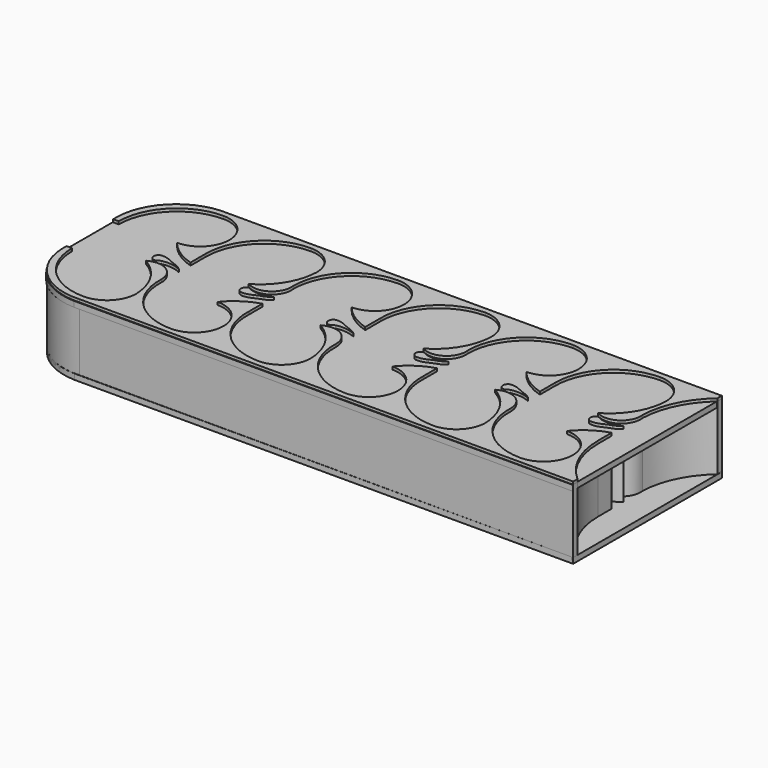
from build123d import *

# Parameters (mm, degrees)
F1_DEPTH = 12
F3_DEPTH = 0.5
F5_DEPTH = 1
F6_DEPTH = 0.5
F7_DEPTH = 0.5


# Not quite as in the source:
# - ends of sketch curves that miss each other by under 0.0002 mm in the source are joined


with BuildPart() as f1:
    # F0 (on Top) → F1 (new body)
    with BuildSketch(Plane.XY):
        with BuildLine():
            Line((-4.0578052044, 17.8321947956), (-3.0578052044, 17.8321947956))
            ThreePointArc((-3.0578052044, 17.8321947956), (0, 25.2143895912), (7.3821947956, 28.2721947956))
            ThreePointArc((7.3821947956, 28.2721947956), (12.6021947956, 23.0521947956), (7.3821947956, 17.8321947956))
            ThreePointArc((7.3821947956, 17.8321947956), (9.7268158019, 15.6873529518), (12.6080603792, 14.3471947956))
            Line((12.6080603792, 14.3471947956), (12.6057125985, 17.8321947956))
            ThreePointArc((12.6057125985, 17.8321947956), (15.663517803, 25.2143895912), (23.0457125985, 28.2721947956))
            ThreePointArc((23.0457125985, 28.2721947956), (26.735512433, 26.74199463), (28.2657125985, 23.0521947956))
            ThreePointArc((28.2657125985, 23.0521947956), (26.7848210646, 18.0226188401), (23.0457125985, 14.3471947956))
            ThreePointArc((23.0457125985, 14.3471947956), (26.7558378252, 14.4434003756), (28.2692304015, 17.8321947956))
            ThreePointArc((28.2692304015, 17.8321947956), (31.3266820271, 25.2140360912), (38.7082304015, 28.2721948435))
            ThreePointArc((38.7082304015, 28.2721948435), (38.7087304015, 28.2721948794), (38.7092304015, 28.2721948914))
            ThreePointArc((38.7092304015, 28.2721948914), (43.9282304015, 23.0521947956), (38.7092304015, 17.8321948914))
            ThreePointArc((38.7092304015, 17.8321948914), (38.7087304015, 17.8321948195), (38.7082304015, 17.8321947956))
            ThreePointArc((38.7082304015, 17.8321947956), (41.0528514078, 15.6873529518), (43.9340959851, 14.3471947956))
            Line((43.9340959851, 14.3471947956), (43.9317482044, 17.8321947956))
            ThreePointArc((43.9317482044, 17.8321947956), (46.989553375, 25.2143896531), (54.3717482044, 28.2721948914))
            ThreePointArc((54.3717482044, 28.2721948914), (58.0616124348, 26.7423520877), (59.5907482044, 23.0521947956))
            ThreePointArc((59.5907482044, 23.0521947956), (58.1098566705, 18.0226188401), (54.3707482044, 14.3471947956))
            ThreePointArc((54.3707482044, 14.3471947956), (58.0808734311, 14.4434003756), (59.5942660074, 17.8321947956))
            ThreePointArc((59.5942660074, 17.8321947956), (62.651717633, 25.2140360912), (70.0332660074, 28.2721948435))
            ThreePointArc((70.0332660074, 28.2721948435), (70.0337660074, 28.2721948794), (70.0342660074, 28.2721948914))
            ThreePointArc((70.0342660074, 28.2721948914), (75.2532660074, 23.0521947956), (70.0342660074, 17.8321948914))
            ThreePointArc((70.0342660074, 17.8321948914), (70.0337660074, 17.8321948195), (70.0332660074, 17.8321947956))
            ThreePointArc((70.0332660074, 17.8321947956), (72.3778870137, 15.6873529518), (75.259131591, 14.3471947956))
            Line((75.259131591, 14.3471947956), (75.2567838104, 17.8321947956))
            ThreePointArc((75.2567838104, 17.8321947956), (78.3145889809, 25.2143896531), (85.6967838104, 28.2721948914))
            ThreePointArc((85.6967838104, 28.2721948914), (89.3869966698, 26.74270065), (90.9157838104, 23.0521947956))
            ThreePointArc((90.9157838104, 23.0521947956), (89.4348922764, 18.0226188401), (85.6957838104, 14.3471947956))
            ThreePointArc((85.6957838104, 14.3471947956), (89.405909037, 14.4434003756), (90.9193016133, 17.8321947956))
            ThreePointArc((90.9193016133, 17.8321947956), (92.3441007337, 23.5750026665), (95.9421947956, 28.2721947956))
            Line((95.9421947956, 28.2721947956), (95.9421947956, 29.2721947956))
            Line((95.9421947956, 29.2721947956), (7.3821947956, 29.2721947956))
            ThreePointArc((7.3821947956, 29.2721947956), (-0.5342205883, 26.4589947948), (-4.0578052044, 18.8321947956))
            Line((-4.0578052044, 18.8321947956), (-4.0578052044, 17.8321947956))
        make_face()
    extrude(amount=F1_DEPTH)


with BuildPart() as f1b:
    # F0 (on Top) → F1, piece 2 (new body)
    with BuildSketch(Plane.XY):
        with BuildLine():
            Line((-3.0578052044, 7.3821947956), (-4.0578052044, 7.3821947956))
            Line((-4.0578052044, 7.3821947956), (-4.0578052044, 6.3821947956))
            ThreePointArc((-4.0578052044, 6.3821947956), (-0.532322416, -1.242525214), (7.3821947956, -4.0578052044))
            Line((7.3821947956, -4.0578052044), (95.9421947956, -4.0578052044))
            Line((95.9421947956, -4.0578052044), (95.9421947956, -3.0578052044))
            ThreePointArc((95.9421947956, -3.0578052044), (92.2352959866, 1.8486137013), (90.9193016133, 7.8554601342))
            Line((90.9193016133, 7.8554601342), (90.9193016133, 10.8671947956))
            ThreePointArc((90.9193016133, 10.8671947956), (88.0393184071, 9.5267247614), (85.6957838104, 7.3821947956))
            ThreePointArc((85.6957838104, 7.3821947956), (90.9157838104, 2.1621947956), (85.6957838104, -3.0578052045))
            ThreePointArc((85.6957838104, -3.0578052045), (85.690917339, -3.0578086106), (85.6860508666, -3.0578097483))
            ThreePointArc((85.6860508666, -3.0578097483), (78.1383828537, 0.1692592999), (75.2567838104, 7.8554601342))
            ThreePointArc((75.2567838104, 7.8554601342), (73.515024019, 10.8702438705), (70.0332660074, 10.8671947956))
            ThreePointArc((70.0332660074, 10.8671947956), (73.7723744735, 7.1917707511), (75.2532660074, 2.1621947956))
            ThreePointArc((75.2532660074, 2.1621947956), (73.7199871381, -1.5314121329), (70.0235330637, -3.0578142782))
            ThreePointArc((70.0235330637, -3.0578142782), (62.4758650508, 0.1692592999), (59.5942660074, 7.8554601342))
            Line((59.5942660074, 7.8554601342), (59.5942660074, 10.8671947956))
            ThreePointArc((59.5942660074, 10.8671947956), (56.7142828012, 9.5267247614), (54.3707482044, 7.3821947956))
            ThreePointArc((54.3707482044, 7.3821947956), (59.5907482044, 2.1621947956), (54.3707482044, -3.0578052044))
            ThreePointArc((54.3707482044, -3.0578052044), (54.3658817331, -3.0578086106), (54.3610152607, -3.0578097483))
            ThreePointArc((54.3610152607, -3.0578097483), (46.8133472478, 0.1692592999), (43.9317482044, 7.8554601342))
            ThreePointArc((43.9317482044, 7.8554601342), (42.1899884131, 10.8702438705), (38.7082304015, 10.8671947956))
            ThreePointArc((38.7082304015, 10.8671947956), (42.4473388676, 7.1917707511), (43.9282304015, 2.1621947956))
            ThreePointArc((43.9282304015, 2.1621947956), (42.3950425449, -1.5315033151), (38.6984974577, -3.0578142782))
            ThreePointArc((38.6984974577, -3.0578142782), (31.1508294449, 0.1692592999), (28.2692304015, 7.8554601342))
            Line((28.2692304015, 7.8554601342), (28.2692304015, 10.8671947956))
            ThreePointArc((28.2692304015, 10.8671947956), (25.3892471953, 9.5267247614), (23.0457125985, 7.3821947956))
            ThreePointArc((23.0457125985, 7.3821947956), (26.7368099963, 5.8532921934), (28.2657125985, 2.1621947956))
            ThreePointArc((28.2657125985, 2.1621947956), (26.7368099963, -1.5289026022), (23.0457125985, -3.0578052044))
            ThreePointArc((23.0457125985, -3.0578052044), (23.0403460829, -3.0578093467), (23.0349795658, -3.0578107304))
            ThreePointArc((23.0349795658, -3.0578107304), (15.487310875, 0.1692583362), (12.6057125985, 7.8554604215))
            ThreePointArc((12.6057125985, 7.8554604215), (10.8639528072, 10.8702441579), (7.3821947956, 10.8671950829))
            ThreePointArc((7.3821947956, 10.8671950829), (11.1213033303, 7.1917709136), (12.6021947956, 2.1621947956))
            ThreePointArc((12.6021947956, 2.1621947956), (11.0722754954, -1.5278859042), (7.3821947956, -3.0578052044))
            ThreePointArc((7.3821947956, -3.0578052044), (0, 0), (-3.0578052044, 7.3821947956))
        make_face()
    extrude(amount=F1_DEPTH)


with BuildPart() as f1c:
    # F0 (on Top) → F1, piece 3 (new body)
    with BuildSketch(Plane.XY):
        with BuildLine():
            ThreePointArc((9.9950144552, 13.0421947956), (9.1526392653, 13.3739527192), (8.2531947956, 13.4771947956))
            ThreePointArc((8.2531947956, 13.4771947956), (7.6380119976, 13.2223777968), (7.3831947956, 12.6071950829))
            ThreePointArc((7.3831947956, 12.6071950829), (7.6380117944, 11.9920119976), (8.2531947956, 11.7371947956))
            ThreePointArc((8.2531947956, 11.7371947956), (8.6734073917, 11.9853047468), (9.1241947956, 12.1721947956))
            ThreePointArc((9.1241947956, 12.1721947956), (10.9028963095, 12.2560700802), (12.6062995437, 11.7371947956))
            ThreePointArc((12.6062995437, 11.7371947956), (11.983253552, 12.2040695598), (11.2720043124, 12.5207442706))
            ThreePointArc((11.2720043124, 12.5207442706), (10.6248880882, 12.7603566825), (9.9950144552, 13.0421947956))
        make_face()
    extrude(amount=F1_DEPTH)


with BuildPart() as f1d:
    # F0 (on Top) → F1, piece 4 (new body)
    with BuildSketch(Plane.XY):
        with BuildLine():
            ThreePointArc((24.7867125985, 13.0421947956), (24.3359251946, 13.2290848443), (23.9157125985, 13.4771947956))
            ThreePointArc((23.9157125985, 13.4771947956), (23.3005296989, 13.2223776952), (23.0457125985, 12.6071947956))
            ThreePointArc((23.0457125985, 12.6071947956), (23.3005296989, 11.992011896), (23.9157125985, 11.7371947956))
            ThreePointArc((23.9157125985, 11.7371947956), (24.8152501168, 11.8404135156), (25.6577125985, 12.1721947956))
            ThreePointArc((25.6577125985, 12.1721947956), (26.2876842061, 12.4540520233), (26.9349016865, 12.6936710042))
            ThreePointArc((26.9349016865, 12.6936710042), (27.6465662844, 13.0102546924), (28.269991237, 13.4771947956))
            ThreePointArc((28.269991237, 13.4771947956), (26.5660143275, 12.9581116528), (24.7867125985, 13.0421947956))
        make_face()
    extrude(amount=F1_DEPTH)


with BuildPart() as f1e:
    # F0 (on Top) → F1, piece 5 (new body)
    with BuildSketch(Plane.XY):
        with BuildLine():
            ThreePointArc((41.3200500611, 13.0421947956), (40.4776748712, 13.3739527192), (39.5782304015, 13.4771947956))
            ThreePointArc((39.5782304015, 13.4771947956), (38.9630475019, 13.2223776952), (38.7082304015, 12.6071947956))
            ThreePointArc((38.7082304015, 12.6071947956), (38.9630475019, 11.992011896), (39.5782304015, 11.7371947956))
            ThreePointArc((39.5782304015, 11.7371947956), (39.9984429976, 11.9853047468), (40.4492304015, 12.1721947956))
            ThreePointArc((40.4492304015, 12.1721947956), (42.2279319155, 12.2560700802), (43.9313351496, 11.7371947956))
            ThreePointArc((43.9313351496, 11.7371947956), (43.3082891579, 12.2040695598), (42.5970399183, 12.5207442706))
            ThreePointArc((42.5970399183, 12.5207442706), (41.9499236941, 12.7603566825), (41.3200500611, 13.0421947956))
        make_face()
    extrude(amount=F1_DEPTH)


with BuildPart() as f1f:
    # F0 (on Top) → F1, piece 6 (new body)
    with BuildSketch(Plane.XY):
        with BuildLine():
            ThreePointArc((56.1117482044, 13.0421947956), (55.6609608006, 13.2290848443), (55.2407482044, 13.4771947956))
            ThreePointArc((55.2407482044, 13.4771947956), (54.6255653048, 13.2223776952), (54.3707482044, 12.6071947956))
            ThreePointArc((54.3707482044, 12.6071947956), (54.6255653048, 11.992011896), (55.2407482044, 11.7371947956))
            ThreePointArc((55.2407482044, 11.7371947956), (56.1402857227, 11.8404135156), (56.9827482044, 12.1721947956))
            ThreePointArc((56.9827482044, 12.1721947956), (57.612719812, 12.4540520233), (58.2599372924, 12.6936710042))
            ThreePointArc((58.2599372924, 12.6936710042), (58.9716018903, 13.0102546924), (59.5950268429, 13.4771947956))
            ThreePointArc((59.5950268429, 13.4771947956), (57.8910499334, 12.9581116528), (56.1117482044, 13.0421947956))
        make_face()
    extrude(amount=F1_DEPTH)


with BuildPart() as f1g:
    # F0 (on Top) → F1, piece 7 (new body)
    with BuildSketch(Plane.XY):
        with BuildLine():
            ThreePointArc((72.645085667, 13.0421947956), (71.8027104771, 13.3739527192), (70.9032660074, 13.4771947956))
            ThreePointArc((70.9032660074, 13.4771947956), (70.2880831078, 13.2223776952), (70.0332660074, 12.6071947956))
            ThreePointArc((70.0332660074, 12.6071947956), (70.2880831078, 11.992011896), (70.9032660074, 11.7371947956))
            ThreePointArc((70.9032660074, 11.7371947956), (71.3234786035, 11.9853047468), (71.7742660074, 12.1721947956))
            ThreePointArc((71.7742660074, 12.1721947956), (73.5529675214, 12.2560700802), (75.2563707555, 11.7371947956))
            ThreePointArc((75.2563707555, 11.7371947956), (74.6333247638, 12.2040695598), (73.9220755242, 12.5207442706))
            ThreePointArc((73.9220755242, 12.5207442706), (73.2749593, 12.7603566825), (72.645085667, 13.0421947956))
        make_face()
    extrude(amount=F1_DEPTH)


with BuildPart() as f1h:
    # F0 (on Top) → F1, piece 8 (new body)
    with BuildSketch(Plane.XY):
        with BuildLine():
            ThreePointArc((87.4367838104, 13.0421947956), (86.9859964065, 13.2290848443), (86.5657838104, 13.4771947956))
            ThreePointArc((86.5657838104, 13.4771947956), (85.9506009107, 13.2223776952), (85.6957838104, 12.6071947956))
            ThreePointArc((85.6957838104, 12.6071947956), (85.9506009107, 11.992011896), (86.5657838104, 11.7371947956))
            ThreePointArc((86.5657838104, 11.7371947956), (87.4653213286, 11.8404135156), (88.3077838104, 12.1721947956))
            ThreePointArc((88.3077838104, 12.1721947956), (88.9377554179, 12.4540520233), (89.5849728984, 12.6936710042))
            ThreePointArc((89.5849728984, 12.6936710042), (90.2966374962, 13.0102546924), (90.9200624488, 13.4771947956))
            ThreePointArc((90.9200624488, 13.4771947956), (89.2160855393, 12.9581116528), (87.4367838104, 13.0421947956))
        make_face()
    extrude(amount=F1_DEPTH)


with BuildPart() as f3:
    # F2 (on Top) → F3 (new body, symmetric)
    with BuildSketch(Plane.XY):
        with BuildLine():
            Line((95.9630012512, 29.2796920985), (6.57434389, 29.2796920985))
            ThreePointArc((6.57434389, 29.2796920985), (-1.1655044994, 25.8072300343), (-4.0526320226, 17.8305301815))
            Line((-4.0526320226, 17.8305301815), (-4.0632681921, 7.387293037))
            ThreePointArc((-4.0632681921, 7.387293037), (-1.1640757991, -0.601379036), (6.57434389, -4.1143633425))
            Line((6.57434389, -4.1143633425), (95.946714282, -4.057593178))
            Line((95.946714282, -4.057593178), (95.9630012512, 29.2796920985))
        make_face()
    extrude(amount=F3_DEPTH, both=True)


with BuildPart() as f5:
    # F4 (on face) → F5 (new body)
    with BuildSketch(Plane.XY.offset(12)):
        with BuildLine():
            ThreePointArc((-4.0578052044, 18.8321947956), (-3.5685461983, 21.6977233687), (-2.3347808732, 24.3299185555))
            ThreePointArc((-2.3347808732, 24.3299185555), (-3.7611187628, 21.1817173411), (-4.1269790381, 17.7448936738))
            Line((-4.1269790381, 17.7448936738), (-4.1376152076, 7.3016565293))
            ThreePointArc((-4.1376152076, 7.3016565293), (-1.2384228146, -0.6870155437), (6.4999968745, -4.1999998502))
            Line((6.4999968745, -4.1999998502), (95.8723672666, -4.1432296857))
            Line((95.8723672666, -4.1432296857), (95.8881809775, 28.2253581749))
            ThreePointArc((95.8881809775, 28.2253581749), (92.3286425892, 23.542771655), (90.9193016133, 17.8321947956))
            ThreePointArc((90.9193016133, 17.8321947956), (89.405909037, 14.4434003756), (85.6957838104, 14.3471947956))
            ThreePointArc((85.6957838104, 14.3471947956), (89.4348922764, 18.0226188401), (90.9157838104, 23.0521947956))
            ThreePointArc((90.9157838104, 23.0521947956), (89.3869966698, 26.74270065), (85.6967838104, 28.2721948914))
            ThreePointArc((85.6967838104, 28.2721948914), (78.3145889809, 25.2143896531), (75.2567838104, 17.8321947956))
            Line((75.2567838104, 17.8321947956), (75.259131591, 14.3471947956))
            ThreePointArc((75.259131591, 14.3471947956), (72.3778870137, 15.6873529518), (70.0332660074, 17.8321947956))
            ThreePointArc((70.0332660074, 17.8321947956), (70.0337660074, 17.8321948195), (70.0342660074, 17.8321948914))
            ThreePointArc((70.0342660074, 17.8321948914), (75.2532660074, 23.0521948914), (70.0342660074, 28.2721948914))
            ThreePointArc((70.0342660074, 28.2721948914), (70.0337660074, 28.2721948794), (70.0332660074, 28.2721948435))
            ThreePointArc((70.0332660074, 28.2721948435), (62.651717633, 25.2140360912), (59.5942660074, 17.8321947956))
            ThreePointArc((59.5942660074, 17.8321947956), (58.0808734311, 14.4434003756), (54.3707482044, 14.3471947956))
            ThreePointArc((54.3707482044, 14.3471947956), (58.1098566705, 18.0226188401), (59.5907482044, 23.0521947956))
            ThreePointArc((59.5907482044, 23.0521947956), (58.0616124348, 26.7423520877), (54.3717482044, 28.2721948914))
            ThreePointArc((54.3717482044, 28.2721948914), (46.989553375, 25.2143896531), (43.9317482044, 17.8321947956))
            Line((43.9317482044, 17.8321947956), (43.9340959851, 14.3471947956))
            ThreePointArc((43.9340959851, 14.3471947956), (41.0528514078, 15.6873529518), (38.7082304015, 17.8321947956))
            ThreePointArc((38.7082304015, 17.8321947956), (38.7087304015, 17.8321948195), (38.7092304015, 17.8321948914))
            ThreePointArc((38.7092304015, 17.8321948914), (43.9282304015, 23.0521948914), (38.7092304015, 28.2721948914))
            ThreePointArc((38.7092304015, 28.2721948914), (38.7087304015, 28.2721948794), (38.7082304015, 28.2721948435))
            ThreePointArc((38.7082304015, 28.2721948435), (31.3266820271, 25.2140360912), (28.2692304015, 17.8321947956))
            ThreePointArc((28.2692304015, 17.8321947956), (26.7558378252, 14.4434003756), (23.0457125985, 14.3471947956))
            ThreePointArc((23.0457125985, 14.3471947956), (26.7848210646, 18.0226188401), (28.2657125985, 23.0521947956))
            ThreePointArc((28.2657125985, 23.0521947956), (26.735512433, 26.74199463), (23.0457125985, 28.2721947956))
            ThreePointArc((23.0457125985, 28.2721947956), (15.663517803, 25.2143895912), (12.6057125985, 17.8321947956))
            Line((12.6057125985, 17.8321947956), (12.6080603792, 14.3471947956))
            ThreePointArc((12.6080603792, 14.3471947956), (9.7268158019, 15.6873529518), (7.3821947956, 17.8321947956))
            ThreePointArc((7.3821947956, 17.8321947956), (12.6021947956, 23.0521947956), (7.3821947956, 28.2721947956))
            ThreePointArc((7.3821947956, 28.2721947956), (0, 25.2143895912), (-3.0578052044, 17.8321947956))
            Line((-3.0578052044, 17.8321947956), (-4.0578052044, 17.8321947956))
            Line((-4.0578052044, 17.8321947956), (-4.0578052044, 18.8321947956))
        make_face()
    extrude(amount=-F5_DEPTH)


with BuildPart() as f6:
    # F6 (new): a face of the model
    f6_faces = [f1.part.faces().sort_by_distance(p)[0] for p in [
        (0.1478437836, 25.7115985865, 12),
    ]]
    extrude(f6_faces, amount=F6_DEPTH)


with BuildPart() as f7:
    # F7 (new): a face of the model
    f7_faces = [f1h.part.faces().sort_by_distance(p)[0] for p in [
        (87.4055384561, 12.5850681474, 12),
    ]]
    extrude(f7_faces, amount=F7_DEPTH)


with BuildPart() as f7b:
    # F7#2 (new): a face of the model
    f7_2_faces = [f1b.part.faces().sort_by_distance(p)[0] for p in [
        (27.2574260697, 9.3613274649, 12),
    ]]
    extrude(f7_2_faces, amount=F7_DEPTH)


with BuildPart() as f7c:
    # F7#3 (new): a face of the model
    f7_3_faces = [f1g.part.faces().sort_by_distance(p)[0] for p in [
        (71.7430080315, 12.6292718802, 12),
    ]]
    extrude(f7_3_faces, amount=F7_DEPTH)


with BuildPart() as f7d:
    # F7#4 (new): a face of the model
    f7_4_faces = [f1f.part.faces().sort_by_distance(p)[0] for p in [
        (56.0805028502, 12.5850681474, 12),
    ]]
    extrude(f7_4_faces, amount=F7_DEPTH)


with BuildPart() as f7e:
    # F7#5 (new): a face of the model
    f7_5_faces = [f1e.part.faces().sort_by_distance(p)[0] for p in [
        (40.4179724256, 12.6292718802, 12),
    ]]
    extrude(f7_5_faces, amount=F7_DEPTH)


with BuildPart() as f7f:
    # F7#6 (new): a face of the model
    f7_6_faces = [f1d.part.faces().sort_by_distance(p)[0] for p in [
        (24.7554672443, 12.5850681474, 12),
    ]]
    extrude(f7_6_faces, amount=F7_DEPTH)


with BuildPart() as f7g:
    # F7#7 (new): a face of the model
    f7_7_faces = [f1c.part.faces().sort_by_distance(p)[0] for p in [
        (9.0929368197, 12.6292718802, 12),
    ]]
    extrude(f7_7_faces, amount=F7_DEPTH)


solid = Compound([f1.part, f1b.part, f1c.part, f1d.part, f1e.part, f1f.part, f1g.part, f1h.part, f3.part, f5.part, f6.part, f7.part, f7b.part, f7c.part, f7d.part, f7e.part, f7f.part, f7g.part])
